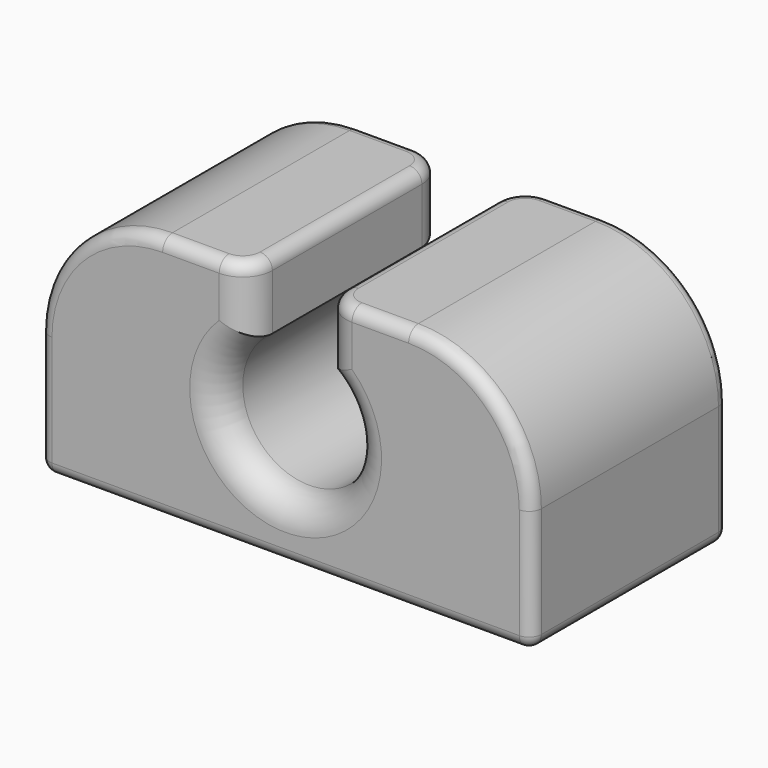
from build123d import *

# Parameters (mm, degrees)
F2_DEPTH = 0.8
F3_DEPTH = 10
F4_R     = 1.2
F5_R     = 5
F6_R     = 0.5


# Not quite as in the source:
# - a feature names something its author has since deleted; it is built from what else it names


with BuildPart() as f2:
    # F1 (on Front) → F2 (new body)
    with BuildSketch(Plane.XZ):
        with BuildLine():
            Line((8.5, 20), (0, 20))
            Line((0, 20), (0, 10))
            Line((0, 10), (20, 10))
            Line((20, 10), (20, 20))
            Line((20, 20), (11.5, 20))
            Line((11.5, 20), (11.5, 17.2449944321))
            ThreePointArc((11.5, 17.2449944321), (10, 12.3), (8.5, 17.2449944321))
            Line((8.5, 17.2449944321), (8.5, 20))
        make_face()
    extrude(amount=F2_DEPTH)

    # F1 (on Front) → F3 (join)
    with BuildSketch(Plane.XZ):
        with BuildLine():
            Line((8.5, 20), (0, 20))
            Line((0, 20), (0, 10))
            Line((0, 10), (20, 10))
            Line((20, 10), (20, 20))
            Line((20, 20), (11.5, 20))
            Line((11.5, 20), (11.5, 17.2449944321))
            ThreePointArc((11.5, 17.2449944321), (10, 12.3), (8.5, 17.2449944321))
            Line((8.5, 17.2449944321), (8.5, 20))
        make_face()
    extrude(amount=F3_DEPTH)

    # F4
    f4_edges = [f2.edges().sort_by_distance(p)[0] for p in [
        (10, -10, 12.3),
        (8.5, -10, 18.622497),
        (11.5, -10, 18.622497),
        (10, 0, 12.3),
        (8.5, 0, 18.622497),
        (11.5, 0, 18.622497),
    ]]
    fillet(f4_edges, radius=F4_R)

    # F5
    f5_edges = [f2.edges().sort_by_distance(p)[0] for p in [
        (20, -5, 20),
        (0, -5, 20),
    ]]
    fillet(f5_edges, radius=F5_R)

    # F6
    f6_edges = [f2.edges().sort_by_distance(p)[0] for p in [
        (1.464466, -10, 18.535534),
        (0, -10, 12.5),
        (10, -10, 10),
        (18.535534, -10, 18.535534),
        (18.535534, 0, 18.535534),
        (1.464466, 0, 18.535534),
        (20, -5, 10),
        (0, -5, 10),
        (10, 0, 10),
    ]]
    fillet(f6_edges, radius=F6_R)


solid = f2.part
